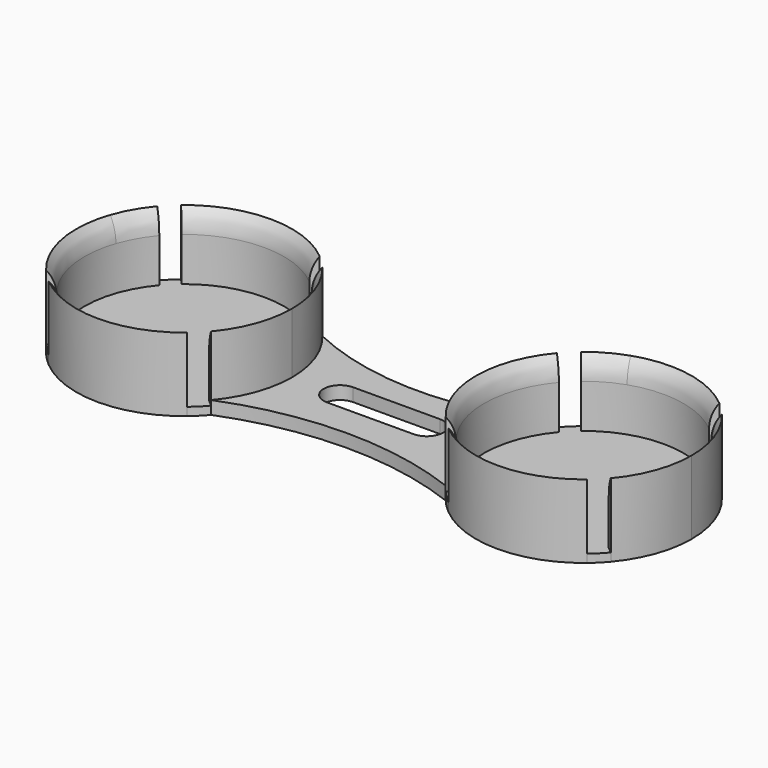
from build123d import *

# Parameters (mm, degrees)
F1_DEPTH      = 1.27
F2_DEPTH      = 11.43
F5_DEPTH      = 1.27
F6_DEPTH      = 11.43
F7_DEPTH      = 2.032
F8_T2_ANGLE   = 142.146924413
F8_T4_ANGLE   = 142.146924413
F8_T6_ANGLE   = 142.146924413
F8_T8_ANGLE   = 142.146924413
F8_2_T2_ANGLE = 142.146924413
F8_2_T4_ANGLE = 142.146924413
F8_2_T6_ANGLE = 142.146924413
F8_2_T8_ANGLE = 142.146924413


# Not quite as in the source:
# - a fillet or chamfer that OpenCascade refuses, or shapes differently, is made with other operations: its cross-section is extruded or revolved along the edge and cut away or added


with BuildPart() as f1:
    # F0 (on Top) → F1 (new body)
    with BuildSketch(Plane.XY):
        with BuildLine():
            Line((-58.8084492598, 23.2332571533), (-57.9905657558, 24.2048365756))
            ThreePointArc((-57.9905657558, 24.2048365756), (-58.9856762328, 25.1195974227), (-59.8972733528, 26.1176069212))
            Line((-59.8972733528, 26.1176069212), (-60.8714443647, 25.3028119534))
            ThreePointArc((-60.8714443647, 25.3028119534), (-59.8851261693, 24.2229983976), (-58.8084492598, 23.2332571533))
        make_face()
        with BuildLine():
            Line((-35.1875386324, 25.262043276), (-36.1591180547, 26.07992678))
            ThreePointArc((-36.1591180547, 26.07992678), (-37.0738789018, 25.0848163031), (-38.0718884004, 24.173219183))
            Line((-38.0718884004, 24.173219183), (-37.2570934326, 23.1990481711))
            ThreePointArc((-37.2570934326, 23.1990481711), (-36.1772798767, 24.1853663666), (-35.1875386324, 25.262043276))
        make_face()
        with BuildLine():
            ThreePointArc((-38.0342082591, 47.9113744811), (-37.0390977822, 46.9966136341), (-36.1275006621, 45.9986041355))
            Line((-36.1275006621, 45.9986041355), (-35.1533296502, 46.8133991033))
            ThreePointArc((-35.1533296502, 46.8133991033), (-36.1396478457, 47.8932126591), (-37.2163247552, 48.8829539035))
            Line((-37.2163247552, 48.8829539035), (-38.0342082591, 47.9113744811))
        make_face()
        with BuildLine():
            ThreePointArc((-59.8656559602, 46.0362842767), (-58.9508951132, 47.0313947536), (-57.9528856146, 47.9429918737))
            Line((-57.9528856146, 47.9429918737), (-58.7676805824, 48.9171628856))
            ThreePointArc((-58.7676805824, 48.9171628856), (-59.8474941382, 47.9308446901), (-60.8372353826, 46.8541677807))
            Line((-60.8372353826, 46.8541677807), (-59.8656559602, 46.0362842767))
        make_face()
        with BuildLine():
            ThreePointArc((-36.1591180547, 26.07992678), (-33.4569999437, 30.7472917091), (-32.5183870075, 36.0581055284))
            ThreePointArc((-32.5183870075, 36.0581055284), (-33.4485883094, 41.3458085725), (-36.1275006621, 45.9986041355))
            ThreePointArc((-36.1275006621, 45.9986041355), (-37.0390977822, 46.9966136341), (-38.0342082591, 47.9113744811))
            ThreePointArc((-38.0342082591, 47.9113744811), (-47.987793042, 51.5520860091), (-57.9528856146, 47.9429918737))
            ThreePointArc((-57.9528856146, 47.9429918737), (-58.9508951132, 47.0313947536), (-59.8656559602, 46.0362842767))
            ThreePointArc((-59.8656559602, 46.0362842767), (-63.5063674882, 36.0826994939), (-59.8972733528, 26.1176069212))
            ThreePointArc((-59.8972733528, 26.1176069212), (-58.9856762328, 25.1195974227), (-57.9905657558, 24.2048365756))
            ThreePointArc((-57.9905657558, 24.2048365756), (-48.036980973, 20.5641250476), (-38.0718884004, 24.173219183))
            ThreePointArc((-38.0718884004, 24.173219183), (-37.0738789018, 25.0848163031), (-36.1591180547, 26.07992678))
        make_face()
    extrude(amount=F1_DEPTH)

    # F0 (on Top) → F2 (join)
    with BuildSketch(Plane.XY):
        with BuildLine():
            ThreePointArc((-59.8972733528, 26.1176069212), (-63.5063674882, 36.0826994939), (-59.8656559602, 46.0362842767))
            Line((-59.8656559602, 46.0362842767), (-60.8372353826, 46.8541677807))
            ThreePointArc((-60.8372353826, 46.8541677807), (-64.7763658883, 36.0847153927), (-60.8714443647, 25.3028119534))
            Line((-60.8714443647, 25.3028119534), (-59.8972733528, 26.1176069212))
        make_face()
        with BuildLine():
            ThreePointArc((-57.9528856146, 47.9429918737), (-47.987793042, 51.5520860091), (-38.0342082591, 47.9113744811))
            Line((-38.0342082591, 47.9113744811), (-37.2163247552, 48.8829539035))
            ThreePointArc((-37.2163247552, 48.8829539035), (-47.9857771431, 52.8220844091), (-58.7676805824, 48.9171628856))
            Line((-58.7676805824, 48.9171628856), (-57.9528856146, 47.9429918737))
        make_face()
        with BuildLine():
            ThreePointArc((-36.1275006621, 45.9986041355), (-33.4485883094, 41.3458085725), (-32.5183870075, 36.0581055284))
            ThreePointArc((-32.5183870075, 36.0581055284), (-33.4569999437, 30.7472917091), (-36.1591180547, 26.07992678))
            Line((-36.1591180547, 26.07992678), (-35.1875386324, 25.262043276))
            ThreePointArc((-35.1875386324, 25.262043276), (-32.2639354303, 30.3119791009), (-31.2483870075, 36.0581055284))
            ThreePointArc((-31.2483870075, 36.0581055284), (-32.2548343178, 41.7792268548), (-35.1533296502, 46.8133991033))
            Line((-35.1533296502, 46.8133991033), (-36.1275006621, 45.9986041355))
        make_face()
        with BuildLine():
            Line((-37.2570934326, 23.1990481711), (-38.0718884004, 24.173219183))
            ThreePointArc((-38.0718884004, 24.173219183), (-48.036980973, 20.5641250476), (-57.9905657558, 24.2048365756))
            Line((-57.9905657558, 24.2048365756), (-58.8084492598, 23.2332571533))
            ThreePointArc((-58.8084492598, 23.2332571533), (-48.0389968718, 19.2941266476), (-37.2570934326, 23.1990481711))
        make_face()
    extrude(amount=F2_DEPTH)


with BuildPart() as f3_1:
    # F3: copy of F1
    add(f1.part.moved(Location((44.958, 0, 0))))


with BuildPart() as f5:
    # F0 (on Top) → F5 (new body)
    with BuildSketch(Plane.XY):
        with BuildLine():
            ThreePointArc((3.2083194176, 49.0749047633), (2.1285058618, 48.0885865678), (1.1387646174, 47.0119096584))
            Line((1.1387646174, 47.0119096584), (2.1103440398, 46.1940261544))
            ThreePointArc((2.1103440398, 46.1940261544), (-1.5303674882, 36.2404413716), (2.0787266472, 26.2753487989))
            Line((2.0787266472, 26.2753487989), (1.1045556353, 25.4605538311))
            ThreePointArc((1.1045556353, 25.4605538311), (2.0908738307, 24.3807402753), (3.1675507402, 23.3909990309))
            Line((3.1675507402, 23.3909990309), (3.9854342442, 24.3625784533))
            ThreePointArc((3.9854342442, 24.3625784533), (13.939019027, 20.7218669253), (23.9041115996, 24.3309610607))
            Line((23.9041115996, 24.3309610607), (24.7189065674, 23.3567900488))
            ThreePointArc((24.7189065674, 23.3567900488), (25.7987201233, 24.3431082443), (26.7884613676, 25.4197851537))
            Line((26.7884613676, 25.4197851537), (25.8168819453, 26.2376686577))
            ThreePointArc((25.8168819453, 26.2376686577), (29.4575934732, 36.1912534405), (25.8484993379, 46.1563460132))
            Line((25.8484993379, 46.1563460132), (26.8226703498, 46.971140981))
            ThreePointArc((26.8226703498, 46.971140981), (25.8363521543, 48.0509545368), (24.7596752448, 49.0406957811))
            Line((24.7596752448, 49.0406957811), (23.9417917409, 48.0691163588))
            ThreePointArc((23.9417917409, 48.0691163588), (13.988206958, 51.7098278868), (4.0231143854, 48.1007337514))
            Line((4.0231143854, 48.1007337514), (3.2083194176, 49.0749047633))
        make_face()
    extrude(amount=F5_DEPTH)

    # F0 (on Top) → F6 (join)
    with BuildSketch(Plane.XY):
        with BuildLine():
            Line((2.1103440398, 46.1940261544), (1.1387646174, 47.0119096584))
            ThreePointArc((1.1387646174, 47.0119096584), (-2.8003658883, 36.2424572704), (1.1045556353, 25.4605538311))
            Line((1.1045556353, 25.4605538311), (2.0787266472, 26.2753487989))
            ThreePointArc((2.0787266472, 26.2753487989), (-1.5303674882, 36.2404413716), (2.1103440398, 46.1940261544))
        make_face()
        with BuildLine():
            Line((3.9854342442, 24.3625784533), (3.1675507402, 23.3909990309))
            ThreePointArc((3.1675507402, 23.3909990309), (13.9370031282, 19.4518685253), (24.7189065674, 23.3567900488))
            Line((24.7189065674, 23.3567900488), (23.9041115996, 24.3309610607))
            ThreePointArc((23.9041115996, 24.3309610607), (13.939019027, 20.7218669253), (3.9854342442, 24.3625784533))
        make_face()
        with BuildLine():
            ThreePointArc((30.7276129925, 36.215847406), (29.7211656822, 41.9369687324), (26.8226703498, 46.971140981))
            Line((26.8226703498, 46.971140981), (25.8484993379, 46.1563460132))
            ThreePointArc((25.8484993379, 46.1563460132), (29.4575934732, 36.1912534405), (25.8168819453, 26.2376686577))
            Line((25.8168819453, 26.2376686577), (26.7884613676, 25.4197851537))
            ThreePointArc((26.7884613676, 25.4197851537), (29.7120645697, 30.4697209786), (30.7276129925, 36.215847406))
        make_face()
        with BuildLine():
            ThreePointArc((24.7596752448, 49.0406957811), (13.9902228569, 52.9798262868), (3.2083194176, 49.0749047633))
            Line((3.2083194176, 49.0749047633), (4.0231143854, 48.1007337514))
            ThreePointArc((4.0231143854, 48.1007337514), (13.988206958, 51.7098278868), (23.9417917409, 48.0691163588))
            Line((23.9417917409, 48.0691163588), (24.7596752448, 49.0406957811))
        make_face()
    extrude(amount=F6_DEPTH)

    # F8#2: fillet of radius 5.08 on 4 edges, made by hand

    # F8_2_s1 → F8_2_t2 (revolve, cut)
    with BuildSketch(Plane(origin=(1.3238627135, -0.4562944313, 0), x_dir=(0, 0, 1), z_dir=(0.9454191795, -0.3258566786, 0))):
        with BuildLine():
            ThreePointArc((8.0698958349, -23.2952932915), (9.8659470592, -22.9671981727), (11.43, -22.0252932915))
            Line((11.43, -22.0252932915), (11.43, -23.2952932915))
            Line((11.43, -23.2952932915), (8.0698958349, -23.2952932915))
        make_face()
    revolve(axis=Axis((13.9636129925, 36.215847406, 11.43), (0, 0, -1)), revolution_arc=F8_2_T2_ANGLE, mode=Mode.SUBTRACT)

    # F8_2_s3 → F8_2_t4 (revolve, cut)
    with BuildSketch(Plane(origin=(12.639750279, 36.6721418373, 0), x_dir=(0, 0, 1), z_dir=(-0.3258566786, -0.9454191795, 0))):
        with BuildLine():
            ThreePointArc((8.0698958349, 14.0937082117), (9.8659470592, 14.4218033305), (11.43, 15.3637082117))
            Line((11.43, 15.3637082117), (11.43, 14.0937082117))
            Line((11.43, 14.0937082117), (8.0698958349, 14.0937082117))
        make_face()
    revolve(axis=Axis((13.9636129925, 36.215847406, 11.43), (0, 0, -1)), revolution_arc=F8_2_T4_ANGLE, mode=Mode.SUBTRACT)

    # F8_2_s5 → F8_2_t6 (revolve, cut)
    with BuildSketch(Plane(origin=(1.3238627135, -0.4562944313, 0), x_dir=(0, 0, 1), z_dir=(-0.9454191795, 0.3258566786, 0))):
        with BuildLine():
            ThreePointArc((8.0698958349, 54.2832932915), (9.8659470592, 54.6113884103), (11.43, 55.5532932915))
            Line((11.43, 55.5532932915), (11.43, 54.2832932915))
            Line((11.43, 54.2832932915), (8.0698958349, 54.2832932915))
        make_face()
    revolve(axis=Axis((13.9636129925, 36.215847406, 11.43), (0, 0, -1)), revolution_arc=F8_2_T6_ANGLE, mode=Mode.SUBTRACT)

    # F8_2_s7 → F8_2_t8 (revolve, cut)
    with BuildSketch(Plane(origin=(12.639750279, 36.6721418373, 0), x_dir=(0, 0, 1), z_dir=(0.3258566786, 0.9454191795, 0))):
        with BuildLine():
            ThreePointArc((8.0698958349, 16.8942917883), (9.8659470592, 17.2223869071), (11.43, 18.1642917883))
            Line((11.43, 18.1642917883), (11.43, 16.8942917883))
            Line((11.43, 16.8942917883), (8.0698958349, 16.8942917883))
        make_face()
    revolve(axis=Axis((13.9636129925, 36.215847406, 11.43), (0, 0, -1)), revolution_arc=F8_2_T8_ANGLE, mode=Mode.SUBTRACT)


with BuildPart() as f7:
    # F0 (on Top) → F7 (new body)
    with BuildSketch(Plane.XY):
        with BuildLine():
            ThreePointArc((1.1387646174, 47.0119096584), (-16.9848098475, 42.8041563832), (-35.1533296502, 46.8133991033))
            ThreePointArc((-35.1533296502, 46.8133991033), (-32.2548343178, 41.7792268548), (-31.2483870075, 36.0581055284))
            ThreePointArc((-31.2483870075, 36.0581055284), (-32.2639354303, 30.3119791009), (-35.1875386324, 25.262043276))
            ThreePointArc((-35.1875386324, 25.262043276), (-17.0601621266, 28.7746998824), (1.1045556353, 25.4605538311))
            ThreePointArc((1.1045556353, 25.4605538311), (-2.8003658883, 36.2424572704), (1.1387646174, 47.0119096584))
        make_face()
        with BuildLine():
            ThreePointArc((-23.8224443714, 33.5667251542), (-26.3713392507, 36.0977990161), (-23.8402653889, 38.6466938954))
            Line((-23.8402653889, 38.6466938954), (-10.3996630978, 38.6938448171))
            ThreePointArc((-10.3996630978, 38.6938448171), (-7.8507682185, 36.1627709552), (-10.3818420803, 33.6138760759))
            Line((-10.3818420803, 33.6138760759), (-23.8224443714, 33.5667251542))
        make_face(mode=Mode.SUBTRACT)
    extrude(amount=F7_DEPTH)


with BuildPart() as f1_1:
    add(f1.part)

    # F8: fillet of radius 5.08 on 4 edges, made by hand

    # F8_s1 → F8_t2 (revolve, cut)
    with BuildSketch(Plane(origin=(6.0103832874, 17.4381315727, 0), x_dir=(0, 0, 1), z_dir=(-0.3258566786, -0.9454191795, 0))):
        with BuildLine():
            ThreePointArc((8.0698958349, 72.6356060366), (9.8659470592, 72.9637011554), (11.43, 73.9056060366))
            Line((11.43, 73.9056060366), (11.43, 72.6356060366))
            Line((11.43, 72.6356060366), (8.0698958349, 72.6356060366))
        make_face()
    revolve(axis=Axis((-48.0123870075, 36.0581055284, 11.43), (0, 0, -1)), revolution_arc=F8_T2_ANGLE, mode=Mode.SUBTRACT)

    # F8_s3 → F8_t4 (revolve, cut)
    with BuildSketch(Plane(origin=(-54.0227702949, 18.6199739556, 0), x_dir=(0, 0, 1), z_dir=(0.9454191795, -0.3258566786, 0))):
        with BuildLine():
            ThreePointArc((8.0698958349, -2.9508675791), (9.8659470592, -2.6227724603), (11.43, -1.6808675791))
            Line((11.43, -1.6808675791), (11.43, -2.9508675791))
            Line((11.43, -2.9508675791), (8.0698958349, -2.9508675791))
        make_face()
    revolve(axis=Axis((-48.0123870075, 36.0581055284, 11.43), (0, 0, -1)), revolution_arc=F8_T4_ANGLE, mode=Mode.SUBTRACT)

    # F8_s5 → F8_t6 (revolve, cut)
    with BuildSketch(Plane(origin=(-54.0227702949, 18.6199739556, 0), x_dir=(0, 0, 1), z_dir=(-0.9454191795, 0.3258566786, 0))):
        with BuildLine():
            ThreePointArc((8.0698958349, 33.9388675791), (9.8659470592, 34.2669626979), (11.43, 35.2088675791))
            Line((11.43, 35.2088675791), (11.43, 33.9388675791))
            Line((11.43, 33.9388675791), (8.0698958349, 33.9388675791))
        make_face()
    revolve(axis=Axis((-48.0123870075, 36.0581055284, 11.43), (0, 0, -1)), revolution_arc=F8_T6_ANGLE, mode=Mode.SUBTRACT)

    # F8_s7 → F8_t8 (revolve, cut)
    with BuildSketch(Plane(origin=(6.0103832874, 17.4381315727, 0), x_dir=(0, 0, 1), z_dir=(0.3258566786, 0.9454191795, 0))):
        with BuildLine():
            ThreePointArc((8.0698958349, -41.6476060366), (9.8659470592, -41.3195109178), (11.43, -40.3776060366))
            Line((11.43, -40.3776060366), (11.43, -41.6476060366))
            Line((11.43, -41.6476060366), (8.0698958349, -41.6476060366))
        make_face()
    revolve(axis=Axis((-48.0123870075, 36.0581055284, 11.43), (0, 0, -1)), revolution_arc=F8_T8_ANGLE, mode=Mode.SUBTRACT)


solid = Compound([f5.part, f7.part, f1_1.part])
